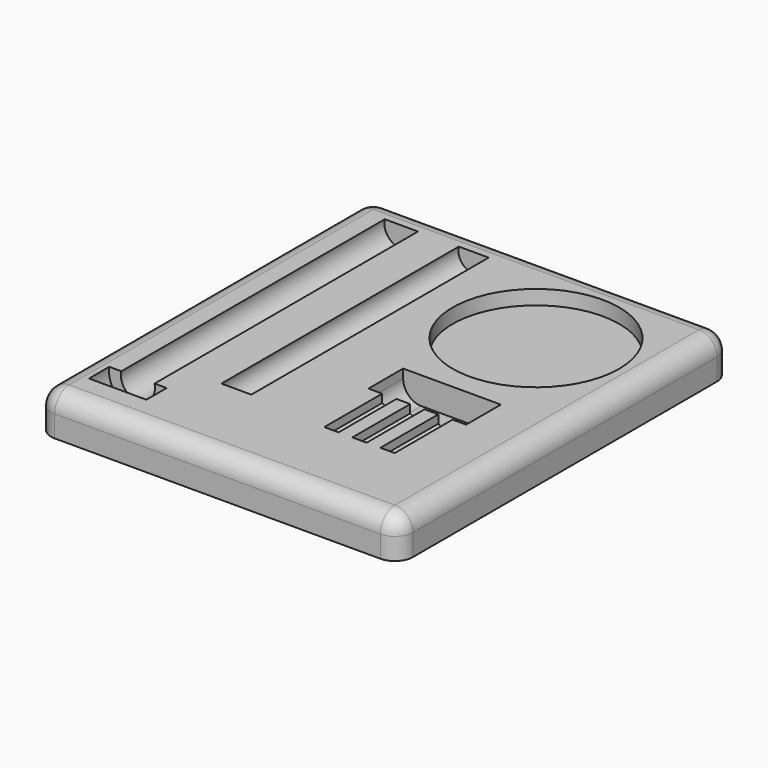
from build123d import *

# Parameters (mm, degrees)
F0_W      = 100
F0_H      = 115
F1_DEPTH  = 15
F2_R      = 23
F3_DEPTH  = 4
F5_R      = 4.7
F6_DEPTH  = 91
F7_R      = 8
F8_DEPTH  = 7
F9_R      = 4.25
F10_DEPTH = 82
F11_W     = 27
F11_H     = 8
F12_DEPTH = 7.5
F14_DEPTH = 20
F15_DEPTH = 4
F16_R     = 5
F17_DEPTH = 4


with BuildPart() as f1:
    # F0 (on Top) → F1 (new body)
    with BuildSketch(Plane.XY):
        with Locations((50, 57.5)):
            Rectangle(F0_W, F0_H)
    extrude(amount=F1_DEPTH)

    # F2 (on face) → F3 (cut)
    with BuildSketch(Plane.XY.offset(15)):
        with Locations((70, 85)):
            Circle(F2_R)
    extrude(amount=-F3_DEPTH, mode=Mode.SUBTRACT)

    # F5 (on offset) → F6 (cut)
    with BuildSketch(Plane(origin=(0, 108, 0), x_dir=(-1, 0, 0), z_dir=(0, 1, 0))):
        with Locations((-14.4, 14)):
            Circle(F5_R)
    extrude(amount=-F6_DEPTH, mode=Mode.SUBTRACT)

    # F7 (on face) → F8 (cut)
    with BuildSketch(Plane(origin=(0, 17, 0), x_dir=(-1, 0, 0), z_dir=(0, 1, 0))):
        with Locations((-14.4, 14)):
            Circle(F7_R)
        with BuildLine():
            ThreePointArc((-9.8076149987, 15), (-14.4, 9.3), (-18.9923850013, 15))
            Line((-18.9923850013, 15), (-9.8076149987, 15))
        make_face(mode=Mode.SUBTRACT)
        with BuildLine():
            Line((-9.8076149987, 15), (-18.9923850013, 15))
            ThreePointArc((-18.9923850013, 15), (-14.4, 9.3), (-9.8076149987, 15))
        make_face()
    extrude(amount=-F8_DEPTH, mode=Mode.SUBTRACT)

    # F9 (on offset) → F10 (cut)
    with BuildSketch(Plane(origin=(0, 108, 0), x_dir=(-1, 0, 0), z_dir=(0, 1, 0))):
        with Locations((-34.4, 14)):
            Circle(F9_R)
    extrude(amount=-F10_DEPTH, mode=Mode.SUBTRACT)

    # F11 (on face) → F12 (cut)
    with BuildSketch(Plane.XY.offset(15)):
        with Locations((70, 48)):
            Rectangle(F11_W, F11_H)
    extrude(amount=-F12_DEPTH, mode=Mode.SUBTRACT)

    # F13 (on face) → F14 (cut)
    with BuildSketch(Plane(origin=(0, 44, 0), x_dir=(-1, 0, 0), z_dir=(0, 1, 0))):
        Polygon((-79.75, 14.9995335633), (-79.75, 12.719), (-77.775, 11.5787332184), (-75.8, 12.719), (-75.8, 14.9995335633), (-75.8008078921, 15), (-79.7491921079, 15), align=None)
        Polygon((-68.0508078921, 15), (-71.9991921079, 15), (-72, 14.9995335633), (-72, 12.719), (-70.025, 11.5787332184), (-68.05, 12.719), (-68.05, 14.9995335633), align=None)
        Polygon((-60.3008078921, 15), (-64.2491921079, 15), (-64.25, 14.9995335633), (-64.25, 12.719), (-62.275, 11.5787332184), (-60.3, 12.719), (-60.3, 14.9995335633), align=None)
    extrude(amount=-F14_DEPTH, mode=Mode.SUBTRACT)

    # F15 (cut): a face of the model
    f15_faces = [f1.faces().sort_by_distance(p)[0] for p in [
        (70, 52, 11.25),
    ]]
    extrude(f15_faces, amount=-F15_DEPTH, mode=Mode.SUBTRACT)

    # F16
    f16_edges = [f1.edges().sort_by_distance(p)[0] for p in [
        (50, 0, 15),
        (100, 57.5, 15),
        (50, 115, 15),
        (0, 57.5, 15),
        (100, 115, 7.5),
        (0, 115, 7.5),
        (100, 0, 7.5),
        (0, 0, 7.5),
        (56.5, 50, 7.5),
        (83.5, 50, 7.5),
    ]]
    fillet(f16_edges, radius=F16_R)

    # F17 (cut): a face of the model
    f17_faces = [f1.faces().sort_by_distance(p)[0] for p in [
        (50, 57.5, 0),
    ]]
    extrude(f17_faces, amount=-F17_DEPTH, mode=Mode.SUBTRACT)


solid = f1.part
